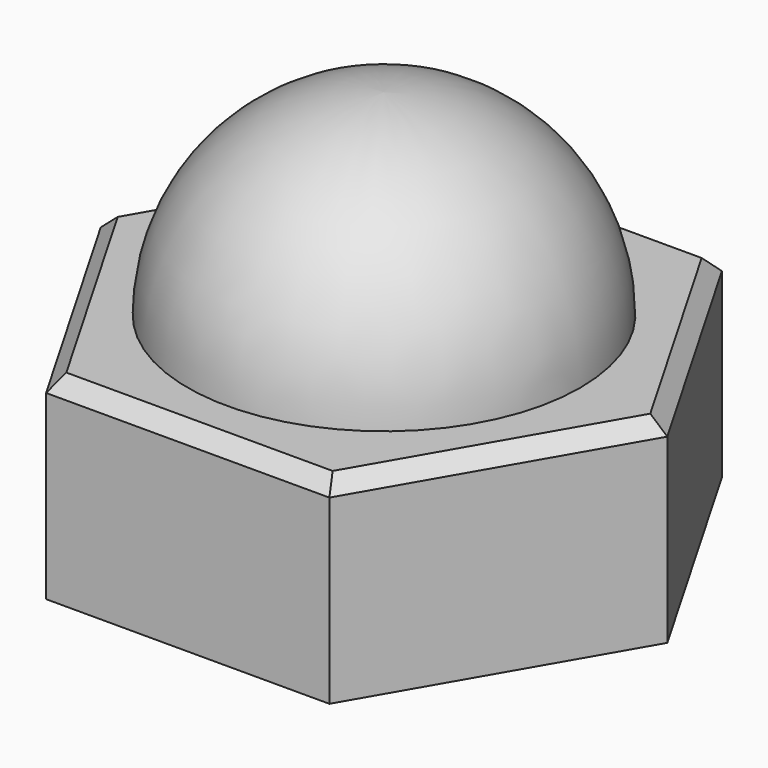
from build123d import *

# Parameters (mm, degrees)
F1_DEPTH = 4
F2_SIZE  = 0.3
F3_R     = 4
F4_DEPTH = 4
F5_R     = 3.99999


# Not quite as in the source:
# - a fillet or chamfer is up to 0.001 mm smaller than in the source, because OpenCascade refuses the exact size


with BuildPart() as f1:
    # F0 (on Top) → F1 (new body)
    with BuildSketch(Plane.XY):
        Polygon((2.8867513459, 5), (-2.8867513459, 5), (-5.7735026919, 0), (-2.8867513459, -5), (2.8867513459, -5), (5.7735026919, 0), align=None)
    extrude(amount=F1_DEPTH)

    # F2
    f2_edges = [f1.edges().sort_by_distance(p)[0] for p in [
        (4.330127, -2.5, 4),
        (0, -5, 4),
        (4.330127, 2.5, 4),
        (-4.330127, -2.5, 4),
        (-4.330127, 2.5, 4),
        (0, 5, 4),
    ]]
    chamfer(f2_edges, length=F2_SIZE)

    # F3 (on face) → F4 (join)
    with BuildSketch(Plane.XY.offset(4)):
        Circle(F3_R)
    extrude(amount=F4_DEPTH)

    # F5 (radius 4 in the source; OpenCascade refuses exactly that, so slightly less here)
    f5_edges = [f1.edges().sort_by_distance(p)[0] for p in [
        (-4, 0, 8),
    ]]
    fillet(f5_edges, radius=F5_R)


solid = f1.part
